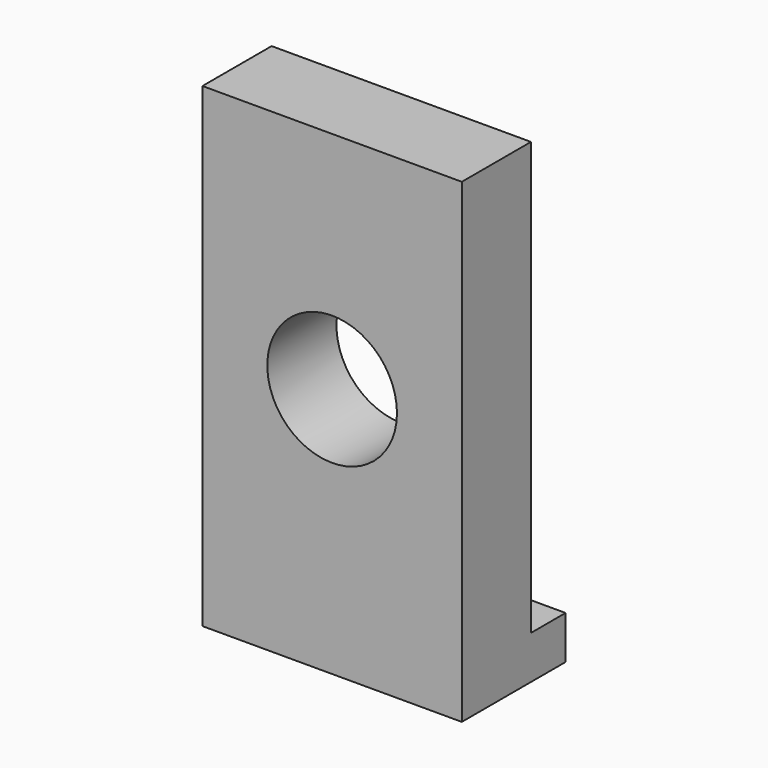
from build123d import *

# Parameters (mm, degrees)
F0_W       = 30
F0_H       = 50
F0_R       = 7.5
F0_H_2     = 5
F1_DEPTH   = 10
F2_W       = 30
F2_H       = 5
F1_FACE1_W = 30
F1_FACE1_H = 55
F1_FACE1_R = 7.5
F3_DEPTH   = 5


# Not quite as in the source:
# - a feature names something its author has since deleted; it is built from what else it names


with BuildPart() as f1:
    # F0 (on Front) → F1 (new body)
    with BuildSketch(Plane.XZ):
        Rectangle(F0_W, F0_H)
        with Locations((0, -1)):
            Circle(F0_R, mode=Mode.SUBTRACT)
        with Locations((0, -27.5)):
            Rectangle(F0_W, F0_H_2)
    extrude(amount=F1_DEPTH)

    # F2 (on face) + F1_face1 (on face) → F3 (join)
    with BuildSketch(Plane(origin=(0, 0, 0), x_dir=(-1, 0, 0), z_dir=(0, 1, 0))):
        with Locations((0, -27.5)):
            Rectangle(F2_W, F2_H)
    with BuildSketch(Plane(origin=(0, -10, -2.6799188927), x_dir=(1, 0, 0), z_dir=(0, -1, 0))):
        with Locations((0, 0.1799188927)):
            Rectangle(F1_FACE1_W, F1_FACE1_H)
        with Locations((0, 1.6799188927)):
            Circle(F1_FACE1_R, mode=Mode.SUBTRACT)
    extrude(amount=F3_DEPTH, dir=(0, 1, 0))


solid = f1.part
